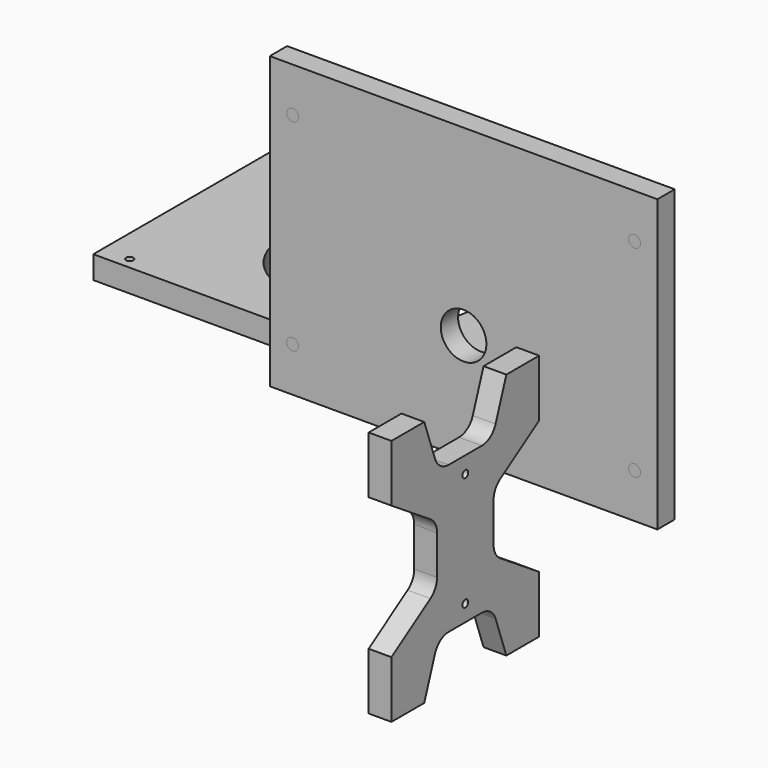
from build123d import *

# Parameters (mm, degrees)
F0_W     = 90
F0_H     = 108.5
F0_R     = 2.6
F0_R_2   = 1.6
F0_R_3   = 35
F0_R_4   = 10
F0_W_2   = 40
F1_DEPTH = 9.5
F2_W     = 170
F2_H     = 100
F2_R     = 1.6
F3_DEPTH = 10
F4_R     = 1.6
F5_DEPTH = 10
F6_DEPTH = 9.5
F7_DEPTH = 9.5


# Not quite as in the source:
# - a feature names something its author has since deleted; it is built from what else it names


with BuildPart() as f1:
    # F0 (on Front) → F1 (new body)
    with BuildSketch(Plane.XZ):
        with Locations((-79.4811890348, 44.25)):
            Rectangle(F0_W, F0_H)
        with Locations((-107.4811890348, 0)):
            Circle(F0_R, mode=Mode.SUBTRACT)
        with Locations((-119.4811890348, 5)):
            Circle(F0_R_2, mode=Mode.SUBTRACT)
        with Locations((-51.4811890348, 0)):
            Circle(F0_R, mode=Mode.SUBTRACT)
        with Locations((-39.4811890348, 5)):
            Circle(F0_R_2, mode=Mode.SUBTRACT)
        with Locations((-79.4811890348, 27.7)):
            Circle(F0_R_3, mode=Mode.SUBTRACT)
        with Locations((-119.4811890348, 83.5)):
            Circle(F0_R_2, mode=Mode.SUBTRACT)
        with Locations((-107.4811890348, 88.5)):
            Circle(F0_R, mode=Mode.SUBTRACT)
        with Locations((-94.4811890348, 78.5)):
            Circle(F0_R, mode=Mode.SUBTRACT)
        with Locations((-64.4811890348, 78.5)):
            Circle(F0_R, mode=Mode.SUBTRACT)
        with Locations((-39.4811890348, 83.5)):
            Circle(F0_R_2, mode=Mode.SUBTRACT)
        with Locations((-51.4811890348, 88.5)):
            Circle(F0_R, mode=Mode.SUBTRACT)
        with Locations((-79.4811890348, 27.7)):
            Circle(F0_R_3)
        with Locations((-104.4811890348, 20)):
            Circle(F0_R, mode=Mode.SUBTRACT)
        with Locations((-79.4811890348, 27.7)):
            Circle(F0_R_4, mode=Mode.SUBTRACT)
        with Locations((-54.4811890348, 20)):
            Circle(F0_R, mode=Mode.SUBTRACT)
        with Locations((-144.4811890348, 44.25)):
            Rectangle(F0_W_2, F0_H)
        with Locations((-154.4811890348, 0)):
            Circle(F0_R, mode=Mode.SUBTRACT)
        with Locations((-154.4374972582, 88.5)):
            Circle(F0_R, mode=Mode.SUBTRACT)
        with Locations((-14.4811890348, 44.25)):
            Rectangle(F0_W_2, F0_H)
        with Locations((-4.4811890348, 0)):
            Circle(F0_R, mode=Mode.SUBTRACT)
        with Locations((-4.4811890348, 88.5)):
            Circle(F0_R, mode=Mode.SUBTRACT)
    extrude(amount=F1_DEPTH)


with BuildPart() as f3:
    # F2 (on Top) → F3 (new body)
    with BuildSketch(Plane.XY):
        with Locations((-164.4811890348, 50)):
            Rectangle(F2_W, F2_H)
        with Locations((-237.4811890348, 5)):
            Circle(F2_R, mode=Mode.SUBTRACT)
        with Locations((-164.4811890348, 5)):
            Circle(F2_R, mode=Mode.SUBTRACT)
        with Locations((-91.4811890348, 5)):
            Circle(F2_R, mode=Mode.SUBTRACT)
        with Locations((-237.4811890348, 95)):
            Circle(F2_R, mode=Mode.SUBTRACT)
        with Locations((-164.4811890348, 95)):
            Circle(F2_R, mode=Mode.SUBTRACT)
        with BuildLine():
            Line((-151.9825607538, 20.4296894372), (-176.9798173157, 20.4296894372))
            ThreePointArc((-176.9798173157, 20.4296894372), (-206.5501278786, 50), (-176.9798173157, 79.5703105628))
            Line((-176.9798173157, 79.5703105628), (-151.9825607538, 79.5703105628))
            ThreePointArc((-151.9825607538, 79.5703105628), (-122.412250191, 50), (-151.9825607538, 20.4296894372))
        make_face(mode=Mode.SUBTRACT)
        with Locations((-91.4811890348, 95)):
            Circle(F2_R, mode=Mode.SUBTRACT)
    extrude(amount=-F3_DEPTH)


with BuildPart() as f5:
    # F4 (on Right) → F5 (new body)
    with BuildSketch(Plane.YZ):
        with BuildLine():
            Line((-142.9015249014, 77.7027970647), (-160.9015249014, 77.7027970647))
            Line((-160.9015249014, 77.7027970647), (-160.9015249014, 52.7027970647))
            Line((-160.9015249014, 52.7027970647), (-139.5289579594, 38.7531395972))
            ThreePointArc((-139.5289579594, 38.7531395972), (-136.8665929353, 35.8630010157), (-135.9015249014, 32.0538367724))
            Line((-135.9015249014, 32.0538367724), (-135.9015249014, 14.851757357))
            ThreePointArc((-135.9015249014, 14.851757357), (-136.8665929353, 11.0425931138), (-139.5289579594, 8.1524545323))
            Line((-139.5289579594, 8.1524545323), (-160.9015249014, -5.7972029353))
            Line((-160.9015249014, -5.7972029353), (-160.9015249014, -30.7972029353))
            Line((-160.9015249014, -30.7972029353), (-142.9015249014, -30.7972029353))
            Line((-142.9015249014, -30.7972029353), (-136.9999515848, -14.1273619005))
            ThreePointArc((-136.9999515848, -14.1273619005), (-134.0760297196, -10.2642584124), (-129.4586023124, -8.7972029353))
            Line((-129.4586023124, -8.7972029353), (-111.3444474904, -8.7972029353))
            ThreePointArc((-111.3444474904, -8.7972029353), (-106.7270200832, -10.2642584124), (-103.8030982179, -14.1273619005))
            Line((-103.8030982179, -14.1273619005), (-97.9015249014, -30.7972029353))
            Line((-97.9015249014, -30.7972029353), (-79.9015249014, -30.7972029353))
            Line((-79.9015249014, -30.7972029353), (-79.9015249014, -5.7972029353))
            Line((-79.9015249014, -5.7972029353), (-101.2740918434, 8.1524545323))
            ThreePointArc((-101.2740918434, 8.1524545323), (-103.9364568675, 11.0425931138), (-104.9015249014, 14.851757357))
            Line((-104.9015249014, 14.851757357), (-104.9015249014, 32.0538367724))
            ThreePointArc((-104.9015249014, 32.0538367724), (-103.9364568675, 35.8630010157), (-101.2740918434, 38.7531395972))
            Line((-101.2740918434, 38.7531395972), (-79.9015249014, 52.7027970647))
            Line((-79.9015249014, 52.7027970647), (-79.9015249014, 77.7027970647))
            Line((-79.9015249014, 77.7027970647), (-97.9015249014, 77.7027970647))
            Line((-97.9015249014, 77.7027970647), (-103.8030982179, 61.03295603))
            ThreePointArc((-103.8030982179, 61.03295603), (-106.7270200832, 57.1698525419), (-111.3444474904, 55.7027970647))
            Line((-111.3444474904, 55.7027970647), (-129.4586023124, 55.7027970647))
            ThreePointArc((-129.4586023124, 55.7027970647), (-134.0760297196, 57.1698525419), (-136.9999515848, 61.03295603))
            Line((-136.9999515848, 61.03295603), (-142.9015249014, 77.7027970647))
        make_face()
        with Locations((-120.4015249014, -1.5472029353)):
            Circle(F4_R, mode=Mode.SUBTRACT)
        with Locations((-120.4015249014, 48.4527970647)):
            Circle(F4_R, mode=Mode.SUBTRACT)
    extrude(amount=F5_DEPTH)


with BuildPart() as f6:
    # F0 (on Front) → F6 (new body)
    with BuildSketch(Plane.XZ):
        with Locations((-79.4811890348, 44.25)):
            Rectangle(F0_W, F0_H)
        with Locations((-107.4811890348, 0)):
            Circle(F0_R, mode=Mode.SUBTRACT)
        with Locations((-119.4811890348, 5)):
            Circle(F0_R_2, mode=Mode.SUBTRACT)
        with Locations((-51.4811890348, 0)):
            Circle(F0_R, mode=Mode.SUBTRACT)
        with Locations((-39.4811890348, 5)):
            Circle(F0_R_2, mode=Mode.SUBTRACT)
        with Locations((-79.4811890348, 27.7)):
            Circle(F0_R_3, mode=Mode.SUBTRACT)
        with Locations((-119.4811890348, 83.5)):
            Circle(F0_R_2, mode=Mode.SUBTRACT)
        with Locations((-107.4811890348, 88.5)):
            Circle(F0_R, mode=Mode.SUBTRACT)
        with Locations((-94.4811890348, 78.5)):
            Circle(F0_R, mode=Mode.SUBTRACT)
        with Locations((-64.4811890348, 78.5)):
            Circle(F0_R, mode=Mode.SUBTRACT)
        with Locations((-39.4811890348, 83.5)):
            Circle(F0_R_2, mode=Mode.SUBTRACT)
        with Locations((-51.4811890348, 88.5)):
            Circle(F0_R, mode=Mode.SUBTRACT)
        with Locations((-51.4811890348, 0)):
            Circle(F0_R)
        with Locations((-14.4811890348, 44.25)):
            Rectangle(F0_W_2, F0_H)
        with Locations((-4.4811890348, 0)):
            Circle(F0_R, mode=Mode.SUBTRACT)
        with Locations((-4.4811890348, 88.5)):
            Circle(F0_R, mode=Mode.SUBTRACT)
        with Locations((-107.4811890348, 0)):
            Circle(F0_R)
        with Locations((-94.4811890348, 78.5)):
            Circle(F0_R)
        with Locations((-64.4811890348, 78.5)):
            Circle(F0_R)
        with Locations((-51.4811890348, 88.5)):
            Circle(F0_R)
        with Locations((-107.4811890348, 88.5)):
            Circle(F0_R)
        with Locations((-144.4811890348, 44.25)):
            Rectangle(F0_W_2, F0_H)
        with Locations((-154.4811890348, 0)):
            Circle(F0_R, mode=Mode.SUBTRACT)
        with Locations((-154.4374972582, 88.5)):
            Circle(F0_R, mode=Mode.SUBTRACT)
        with Locations((-4.4811890348, 88.5)):
            Circle(F0_R)
        with Locations((-4.4811890348, 0)):
            Circle(F0_R)
        with Locations((-154.4811890348, 0)):
            Circle(F0_R)
        with Locations((-154.4374972582, 88.5)):
            Circle(F0_R)
    extrude(amount=F6_DEPTH)


with BuildPart() as f7:
    # F0 (on Front) → F7 (new body)
    with BuildSketch(Plane.XZ):
        with Locations((-144.4811890348, 44.25)):
            Rectangle(F0_W_2, F0_H)
        with Locations((-154.4811890348, 0)):
            Circle(F0_R, mode=Mode.SUBTRACT)
        with Locations((-154.4374972582, 88.5)):
            Circle(F0_R, mode=Mode.SUBTRACT)
        Polygon((-34.4811890348, -10), (-124.4811890348, -10), (-164.4811890348, -10), (-164.4811890348, -19.5), (5.5188109652, -19.5), (5.5188109652, -10), align=None)
        with Locations((-14.4811890348, 44.25)):
            Rectangle(F0_W_2, F0_H)
        with Locations((-4.4811890348, 0)):
            Circle(F0_R, mode=Mode.SUBTRACT)
        with Locations((-4.4811890348, 88.5)):
            Circle(F0_R, mode=Mode.SUBTRACT)
        Polygon((-164.4811890348, 98.5), (-124.4811890348, 98.5), (-34.4811890348, 98.5), (5.5188109652, 98.5), (5.5188109652, 108), (-164.4811890348, 108), align=None)
        with Locations((-79.4811890348, 44.25)):
            Rectangle(F0_W, F0_H)
        with Locations((-107.4811890348, 0)):
            Circle(F0_R, mode=Mode.SUBTRACT)
        with Locations((-119.4811890348, 5)):
            Circle(F0_R_2, mode=Mode.SUBTRACT)
        with Locations((-51.4811890348, 0)):
            Circle(F0_R, mode=Mode.SUBTRACT)
        with Locations((-39.4811890348, 5)):
            Circle(F0_R_2, mode=Mode.SUBTRACT)
        with Locations((-79.4811890348, 27.7)):
            Circle(F0_R_3, mode=Mode.SUBTRACT)
        with Locations((-119.4811890348, 83.5)):
            Circle(F0_R_2, mode=Mode.SUBTRACT)
        with Locations((-107.4811890348, 88.5)):
            Circle(F0_R, mode=Mode.SUBTRACT)
        with Locations((-94.4811890348, 78.5)):
            Circle(F0_R, mode=Mode.SUBTRACT)
        with Locations((-64.4811890348, 78.5)):
            Circle(F0_R, mode=Mode.SUBTRACT)
        with Locations((-39.4811890348, 83.5)):
            Circle(F0_R_2, mode=Mode.SUBTRACT)
        with Locations((-51.4811890348, 88.5)):
            Circle(F0_R, mode=Mode.SUBTRACT)
        with Locations((-79.4811890348, 27.7)):
            Circle(F0_R_3)
        with Locations((-104.4811890348, 20)):
            Circle(F0_R, mode=Mode.SUBTRACT)
        with Locations((-79.4811890348, 27.7)):
            Circle(F0_R_4, mode=Mode.SUBTRACT)
        with Locations((-54.4811890348, 20)):
            Circle(F0_R, mode=Mode.SUBTRACT)
        with Locations((-51.4811890348, 0)):
            Circle(F0_R)
        with Locations((-54.4811890348, 20)):
            Circle(F0_R)
        with Locations((-104.4811890348, 20)):
            Circle(F0_R)
        with Locations((-107.4811890348, 0)):
            Circle(F0_R)
        with Locations((-119.4811890348, 5)):
            Circle(F0_R_2)
        with Locations((-51.4811890348, 88.5)):
            Circle(F0_R)
        with Locations((-64.4811890348, 78.5)):
            Circle(F0_R)
        with Locations((-94.4811890348, 78.5)):
            Circle(F0_R)
        with Locations((-107.4811890348, 88.5)):
            Circle(F0_R)
        with Locations((-119.4811890348, 83.5)):
            Circle(F0_R_2)
        with Locations((-39.4811890348, 83.5)):
            Circle(F0_R_2)
        with Locations((-39.4811890348, 5)):
            Circle(F0_R_2)
    extrude(amount=F7_DEPTH)


solid = Compound([f1.part, f3.part, f5.part, f6.part, f7.part])
